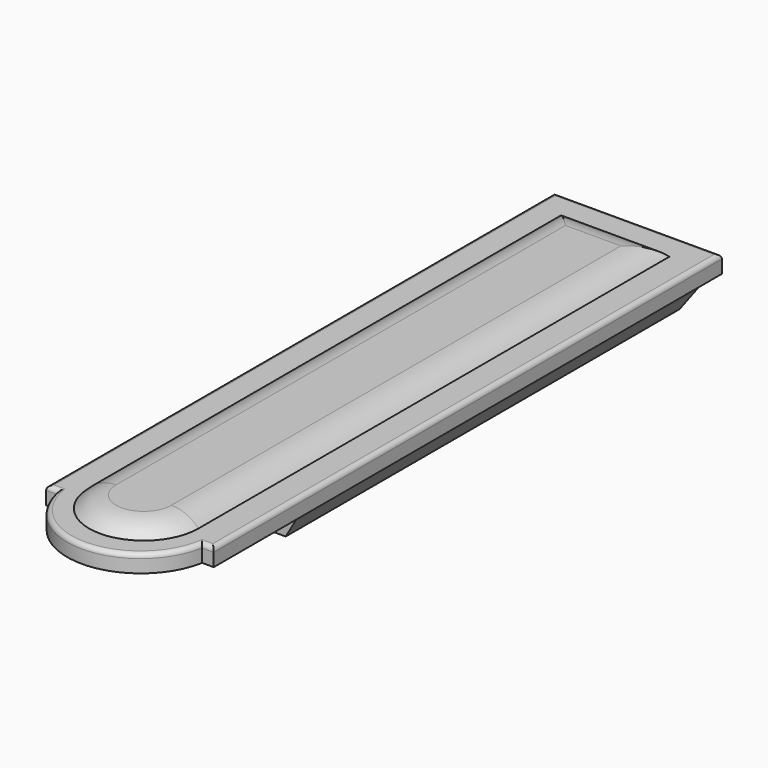
from build123d import *

# Parameters (mm, degrees)
F1_DEPTH    = 3
F3_DEPTH    = 5
F4_SIZE2    = 3.4641016151
F4_SIZE     = 2
F6_DEPTH    = 2
F6_TAPER    = 25
F7_T1_DEPTH = 109.1731798991
F7_T3_DEPTH = 35.3291597983
F7_T6_ANGLE = 180
F8_R        = 0.762


# Not quite as in the source:
# - a fillet or chamfer that OpenCascade refuses, or shapes differently, is made with other operations: its cross-section is extruded or revolved along the edge and cut away or added


with BuildPart() as f1:
    # F0 (on Top) → F1 (new body)
    with BuildSketch(Plane.XY):
        with BuildLine():
            Line((28.7274, 108.839), (0, 108.839))
            Line((0, 108.839), (0, 0))
            Line((0, 0), (1.9812, 0))
            ThreePointArc((1.9812, 0), (14.3637, -10.287), (26.7462, 0))
            Line((26.7462, 0), (28.7274, 0))
            Line((28.7274, 0), (28.7274, 108.839))
        make_face()
    extrude(amount=F1_DEPTH)

    # F2 (on face) → F3 (join)
    with BuildSketch(Plane(origin=(0, 0, 0), x_dir=(1, 0, 0), z_dir=(0, 0, -1))):
        Polygon((6.032, -20.447), (2.032, -20.447), (2.032, -106.807), (26.6954, -106.807), (26.6954, -20.447), (22.6954, -20.447), (22.6954, -102.807), (6.032, -102.807), align=None)
    extrude(amount=F3_DEPTH)

    # F4
    f4_edges = [f1.edges().sort_by_distance(p)[0] for p in [
        (2.032, 63.627, -5),
        (14.3637, 106.807, -5),
        (26.6954, 63.627, -5),
    ]]
    f4_side = f1.faces().sort_by_distance((4.032, 21.345128, -5))[0]
    chamfer(f4_edges, length=F4_SIZE, length2=F4_SIZE2, reference=f4_side)

    # F5 (on face) → F6 (join)
    with BuildSketch(Plane.XY.offset(3)):
        with BuildLine():
            Line((23.7274, 103.839), (5, 103.839))
            Line((5, 103.839), (5, 2.9667))
            ThreePointArc((5, 2.9667), (14.3637, -6.397), (23.7274, 2.9667))
            Line((23.7274, 2.9667), (23.7274, 103.839))
        make_face()
    extrude(amount=F6_DEPTH, taper=F6_TAPER)

    # F7: fillet of radius 6.35 on 4 edges, made by hand

    # F7_s2 → F7_t1 (cut)
    with BuildSketch(Plane.XZ.offset(-112.1398798991)):
        with BuildLine():
            ThreePointArc((23.7274, 3), (21.6213072312, 4.4785933123), (19.1013865975, 5))
            Line((19.1013865975, 5), (22.7947846837, 5))
            Line((22.7947846837, 5), (23.7274, 3))
        make_face()
        with BuildLine():
            ThreePointArc((5, 3), (7.1060927688, 4.4785933123), (9.6260134025, 5))
            Line((9.6260134025, 5), (5.9326153163, 5))
            Line((5.9326153163, 5), (5, 3))
        make_face()
    extrude(amount=F7_T1_DEPTH, mode=Mode.SUBTRACT)

    # F7_s4 → F7_t3 (cut)
    with BuildSketch(Plane.YZ.offset(-3.3008798991)):
        with BuildLine():
            ThreePointArc((103.839, 3), (101.7329072312, 4.4785933123), (99.2129865975, 5))
            Line((99.2129865975, 5), (102.9063846837, 5))
            Line((102.9063846837, 5), (103.839, 3))
        make_face()
    extrude(amount=F7_T3_DEPTH, mode=Mode.SUBTRACT)

    # F7_s5 → F7_t6 (revolve, cut)
    with BuildSketch(Plane.XZ.offset(-2.9667)):
        with BuildLine():
            ThreePointArc((5, 3), (7.1060927688, 4.4785933123), (9.6260134025, 5))
            Line((9.6260134025, 5), (5.9326153163, 5))
            Line((5.9326153163, 5), (5, 3))
        make_face()
    revolve(axis=Axis((14.3637, 2.9667, 5), (0, 0, 1)), revolution_arc=F7_T6_ANGLE, mode=Mode.SUBTRACT)

    # F8
    f8_edges = [f1.edges().sort_by_distance(p)[0] for p in [
        (0, 54.4195, 3),
        (0.9906, 0, 3),
        (14.3637, -10.287, 3),
        (27.7368, 0, 3),
        (28.7274, 54.4195, 3),
        (14.3637, 108.839, 3),
    ]]
    fillet(f8_edges, radius=F8_R)


solid = f1.part
